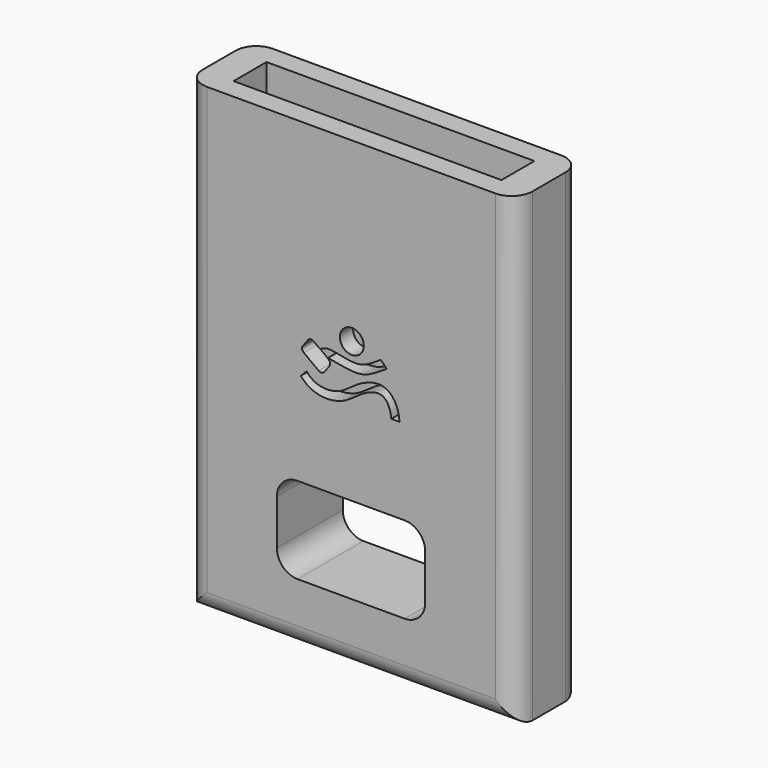
from build123d import *

# Parameters (mm, degrees)
F0_W     = 80
F0_H     = 113
F0_W_2   = 36
F0_H_2   = 21
F1_DEPTH = 20
F3_W     = 65
F3_H     = 10
F4_DEPTH = 65
F6_R     = 2.9
F7_DEPTH = 4
F8_R     = 5


# Not quite as in the source:
# - ends of sketch curves that miss each other by under 0.0002 mm in the source are joined
# - the dataset's text gives a spline's control points without its knots; the knots are read off the source's solid


with BuildPart() as f1:
    # F0 (on Front) → F1 (new body)
    with BuildSketch(Plane.XZ):
        with Locations((-40, 56.5)):
            Rectangle(F0_W, F0_H)
        with Locations((-40, 25.5)):
            Rectangle(F0_W_2, F0_H_2, mode=Mode.SUBTRACT)
    extrude(amount=F1_DEPTH)

    # F3 (on offset) → F4 (cut)
    with BuildSketch(Plane.XY.offset(113)):
        with Locations((-40, -10)):
            Rectangle(F3_W, F3_H)
    extrude(amount=-F4_DEPTH, mode=Mode.SUBTRACT)

    # F6 (on offset) → F7 (cut)
    with BuildSketch(Plane.XZ.offset(20)):
        with BuildLine():
            Line((-45.6861734387, 64.5728954929), (-47.554082421, 65.9506385177))
            Line((-47.554082421, 65.9506385177), (-49.0865064036, 67.0809325915))
            ThreePointArc((-49.0865064036, 67.0809325915), (-49.8294222498, 67.2649502077), (-50.4848631869, 66.8697494794))
            Line((-50.4848631869, 66.8697494794), (-51.672036858, 65.2602095841))
            ThreePointArc((-51.672036858, 65.2602095841), (-51.8560544743, 64.5172937379), (-51.4608537459, 63.8618528009))
            Line((-51.4608537459, 63.8618528009), (-47.8393889815, 61.1907120408))
            ThreePointArc((-47.8393889815, 61.1907120408), (-47.0964731353, 61.0066944245), (-46.4410321982, 61.4018951529))
            Line((-46.4410321982, 61.4018951529), (-45.2538585271, 63.0114350482))
            ThreePointArc((-45.2538585271, 63.0114350482), (-45.0698409108, 63.7543508944), (-45.4650416392, 64.4097918314))
            Line((-45.4650416392, 64.4097918314), (-45.6861734387, 64.5728954929))
        make_face()
        with BuildLine():
            add(Edge.make_bspline(
                [(-47.554082421, 65.9506385177), (-46.8202303366, 66.207397933), (-45.6503607613, 67.2477320434), (-37.8881203208, 64.5849438622), (-35.2091112415, 66.9307097903), (-32.7482156982, 68.4231322687)],
                knots=[0.0446246746, 0.0446246746, 0.0446246746, 0.0446246746, 0.2260814029, 0.5997457356, 0.9327958207, 0.9327958207, 0.9327958207, 0.9327958207], degree=3))
            Line((-47.554082421, 65.9506385177), (-45.6861734387, 64.5728954929))
            add(Edge.make_bspline(
                [(-45.6861734387, 64.5728954929), (-45.6659804328, 64.5796793403), (-45.6378996944, 64.5874559308), (-45.6019050905, 64.5951017149), (-45.5602175432, 64.6009356408), (-45.4994778591, 64.6053291967), (-45.3878563259, 64.6060910244), (-45.2388220323, 64.5994192842), (-44.9963687521, 64.5792423041), (-44.6247938151, 64.5320841175), (-44.0974006097, 64.444859697), (-43.3110890767, 64.2981285875), (-42.2099255417, 64.0792150798), (-41.0220182419, 63.8731448486), (-40.0451032761, 63.7549799735), (-39.3017530405, 63.7012743139), (-38.6735618076, 63.6968929203), (-38.1639179498, 63.7279564894), (-37.4175125658, 63.810141224), (-36.3583666524, 64.0668449543), (-35.1171416014, 64.615286988), (-33.9940206313, 65.2693474202), (-32.8756012123, 65.9875480772), (-31.9714098116, 66.558919637), (-31.4240871624, 66.8856451657), (-31.3280777421, 66.9423467898)],
                knots=[0.1673859512, 0.1673859512, 0.1673859512, 0.1673859512, 0.1875, 0.203125, 0.21875, 0.234375, 0.25, 0.265625, 0.28125, 0.3125, 0.34375, 0.375, 0.4375, 0.5, 0.53125, 0.5625, 0.59375, 0.609375, 0.625, 0.6875, 0.75, 0.8125, 0.875, 0.9375, 0.9505095999, 0.9505095999, 0.9505095999, 0.9505095999], degree=3))
            Line((-31.3280777421, 66.9423467898), (-32.7482156982, 68.4231322687))
        make_face()
        with BuildLine():
            add(Edge.make_bspline(
                [(-50.791586617, 60.1193825298), (-48.7565155629, 57.5566149717), (-42.9029161871, 57.5478755645), (-39.3627682085, 61.1681058444), (-31.8984191451, 64.6120783355), (-28.5156729549, 60.3096565407), (-28.2262380403, 56.6350931128)],
                knots=[0, 0, 0, 0, 0.2652521633, 0.4846441399, 0.7345654281, 1, 1, 1, 1], degree=3))
            Line((-50.791586617, 60.1193825298), (-52.1955544368, 58.6775958054))
            add(Edge.make_bspline(
                [(-52.1955544368, 58.6775958054), (-51.9269511797, 58.3599684), (-51.2960572774, 57.72114106), (-50.2183057784, 56.9486947372), (-49.009380478, 56.3736302806), (-47.3709182638, 55.9019043403), (-45.3654451802, 55.7861788459), (-43.5579128933, 56.0996928302), (-42.2778459687, 56.5281912931), (-41.1311421102, 57.0507932003), (-39.9366678623, 57.813426453), (-38.7482188017, 58.7130941814), (-37.5936622749, 59.5254680789), (-36.2250815272, 60.2913515275), (-35.0500858742, 60.7599425211), (-34.1788245729, 60.9751255859), (-33.5867893323, 61.0501497666), (-33.0777005935, 61.0399467048), (-32.6686463792, 60.9596552649), (-32.2808975454, 60.8046457888), (-31.7796837672, 60.4849491781), (-31.1621676625, 59.8253717032), (-30.5416176329, 58.5207823549), (-30.2959177867, 57.3022437614), (-30.233578431, 56.6350926601)],
                knots=[0.0052987752, 0.0052987752, 0.0052987752, 0.0052987752, 0.03125, 0.0625, 0.09375, 0.125, 0.1875, 0.25, 0.28125, 0.3125, 0.375, 0.4375, 0.5, 0.5625, 0.625, 0.65625, 0.6875, 0.71875, 0.75, 0.78125, 0.8125, 0.875, 0.9375, 0.9954919092, 0.9954919092, 0.9954919092, 0.9954919092], degree=3))
            Line((-30.233578431, 56.6350926601), (-28.2262380403, 56.6350931128))
        make_face()
        with Locations((-39.806915722, 70.0642243504)):
            Circle(F6_R)
    extrude(amount=-F7_DEPTH, mode=Mode.SUBTRACT)

    # F8
    f8_edges = [f1.edges().sort_by_distance(p)[0] for p in [
        (-58, -10, 36),
        (-22, -10, 36),
        (-58, -10, 15),
        (-22, -10, 15),
        (-72.5, -10, 48),
        (-7.5, -10, 48),
        (0, 0, 56.5),
        (0, -20, 56.5),
        (-80, 0, 56.5),
        (-80, -20, 56.5),
        (-40, 0, 0),
        (-40, -20, 0),
    ]]
    fillet(f8_edges, radius=F8_R)


solid = f1.part
